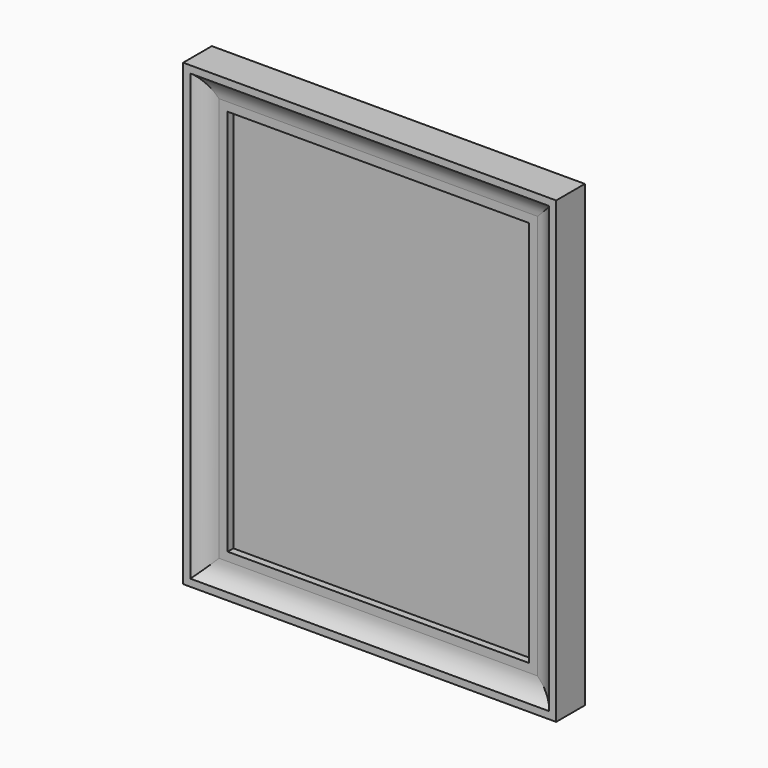
from build123d import *

# Parameters (mm, degrees)
F0_W     = 279.4
F0_H     = 355.6
F1_DEPTH = 9.525
F2_W     = 330.2
F2_H     = 406.4
F2_W_2   = 279.4
F2_H_2   = 355.6
F2_W_3   = 266.7
F2_H_3   = 342.9
F3_DEPTH = 15.875
F4_W     = 330.2
F4_H     = 406.4
F4_W_2   = 279.4
F4_H_2   = 355.6
F5_DEPTH = 15.875


with BuildPart() as f1:
    # F0 (on Front) → F1 (new body)
    with BuildSketch(Plane.XZ):
        Rectangle(F0_W, F0_H)
    extrude(amount=F1_DEPTH)


with BuildPart() as f3:
    # F2 (on face) → F3 (new body)
    with BuildSketch(Plane.XZ.offset(9.525)):
        Rectangle(F2_W, F2_H)
        Rectangle(F2_W_2, F2_H_2, mode=Mode.SUBTRACT)
        Rectangle(F2_W_2, F2_H_2)
        Rectangle(F2_W_3, F2_H_3, mode=Mode.SUBTRACT)
    extrude(amount=F3_DEPTH)

    # F4 (on face) → F5 (join)
    with BuildSketch(Plane(origin=(0, -9.525, 0), x_dir=(-1, 0, 0), z_dir=(0, 1, 0))):
        Rectangle(F4_W, F4_H)
        Rectangle(F4_W_2, F4_H_2, mode=Mode.SUBTRACT)
    extrude(amount=F5_DEPTH)

    # F7: sweep along a path in F7_path
    with BuildLine(Plane(origin=(-133.35, -25.4, -171.45), x_dir=(0, 0, 1), z_dir=(0, -1, 0))) as f7_path:
        Line((0, 0), (342.9, 0))
        Line((342.9, 0), (342.9, -266.7))
        Line((342.9, -266.7), (0, -266.7))
        Line((0, -266.7), (0, 0))
    # F6 (on Top) → F7 (sweep, cut)
    with BuildSketch(Plane.XY):
        with BuildLine():
            Line((-158.75, -25.4), (-133.35, -25.4))
            Line((-133.35, -25.4), (-133.35, -15.875))
            Line((-133.35, -15.875), (-140.97, -15.875))
            ThreePointArc((-140.97, -15.875), (-151.0553114107, -18.4062520334), (-158.75, -25.4))
        make_face()
    sweep(path=f7_path.line, transition=Transition.RIGHT, mode=Mode.SUBTRACT)


solid = Compound([f1.part, f3.part])
